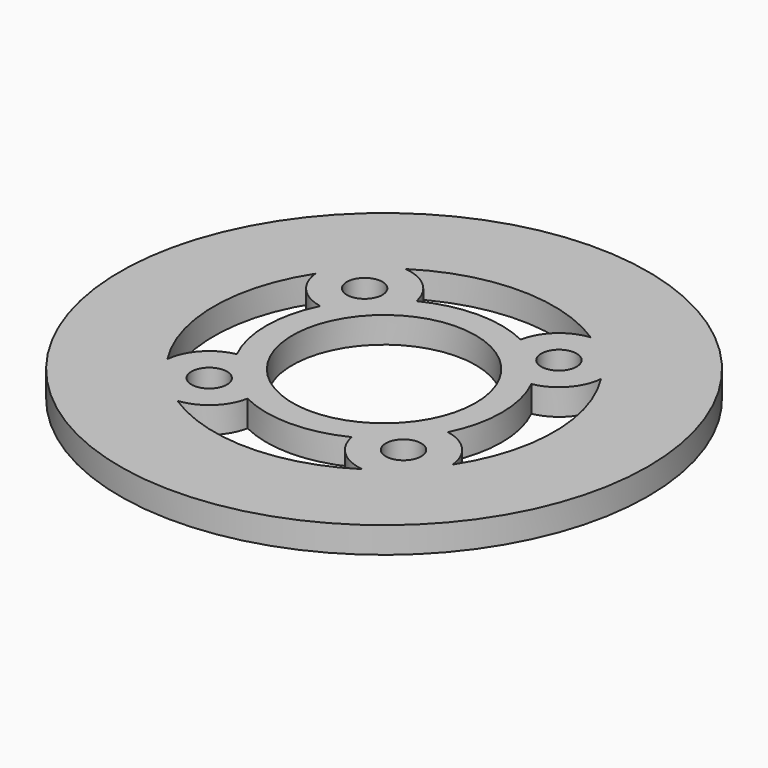
from build123d import *

# Parameters (mm, degrees)
F0_R            = 32.0294
F0_R_2          = 2.15265
F0_R_3          = 11.1125
F1_DEPTH        = 3.175
F3_DEPTH        = 3.175
F3_COPIES_COUNT = 4


# Not quite as in the source:
# - a pattern or mirror of a feature is missing from the dataset's text; its kind, count and spacing are read off the source's solid
# - a feature names something its author has since deleted; it is built from what else it names


with BuildPart() as f1:
    # F0 (on Top) → F1 (new body)
    with BuildSketch(Plane.XY):
        Circle(F0_R)
        with Locations((-11.7865861589, -11.7865861589)):
            Circle(F0_R_2, mode=Mode.SUBTRACT)
        with Locations((11.7865861589, -11.7865861589)):
            Circle(F0_R_2, mode=Mode.SUBTRACT)
        with Locations((-11.7865861589, 11.7865861589)):
            Circle(F0_R_2, mode=Mode.SUBTRACT)
        Circle(F0_R_3, mode=Mode.SUBTRACT)
        with Locations((11.7865861589, 11.7865861589)):
            Circle(F0_R_2, mode=Mode.SUBTRACT)
    extrude(amount=F1_DEPTH)

    # F2 (on face) → F3 (cut, through all)
    with BuildSketch(Plane.XY.offset(3.175)):
        with BuildLine():
            ThreePointArc((-11.229543123, 17.3148424047), (-8.0281867, 15.8788163052), (-6.3255746232, 12.8109235396))
            ThreePointArc((-6.3255746232, 12.8109235396), (0, 14.2875), (6.3255746232, 12.8109235396))
            ThreePointArc((6.3255746232, 12.8109235396), (8.0281867, 15.8788163052), (11.229543123, 17.3148424047))
            ThreePointArc((11.229543123, 17.3148424047), (0, 20.6375), (-11.229543123, 17.3148424047))
        make_face()
    f3 = extrude(amount=-F3_DEPTH, mode=Mode.SUBTRACT)

    # F3_copies: F3 ×4 about axis
    f3_copies_axis = Axis((0, 0, 0), (0, 0, 1))
    for i in range(1, F3_COPIES_COUNT):
        add(f3.rotate(f3_copies_axis, i * 360 / F3_COPIES_COUNT), mode=Mode.SUBTRACT)


solid = f1.part
